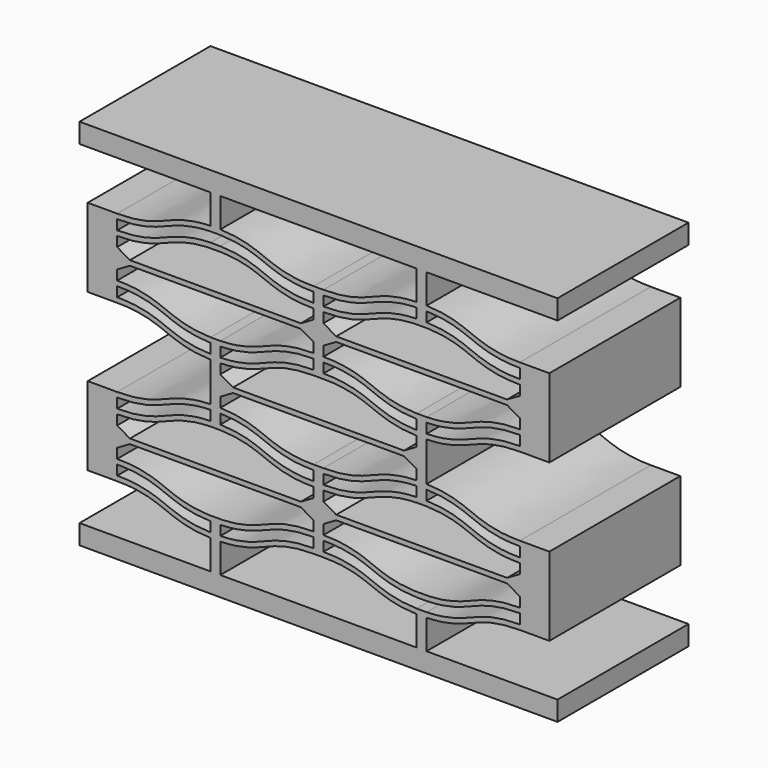
from build123d import *

# Parameters (mm, degrees)
F1_DEPTH = 25


with BuildPart() as f1:
    # F0 (on Front) → F1 (new body)
    with BuildSketch(Plane.XZ):
        with BuildLine():
            add(Edge.make_bspline(
                [(0, 0), (-3.75, 0), (-7.3706402366, -1.4482560946), (-10.9912804731, -2.8965121892), (-14.25, -2.9895365677)],
                knots=[0, 0, 0, 0, 0.5, 0.9655040631, 0.9655040631, 0.9655040631, 0.9655040631], degree=3))
            Line((0, 0), (1.5, 0))
            add(Edge.make_bspline(
                [(15.75, -2.9895365677), (12.4912804731, -2.8965121892), (8.8706402366, -1.4482560946), (5.25, 0), (1.5, 0)],
                knots=[0.0344959369, 0.0344959369, 0.0344959369, 0.0344959369, 0.5, 1, 1, 1, 1], degree=3))
            add(Edge.make_bspline(
                [(16.5, -3), (16.2412804731, -3), (15.9914857187, -2.996430091), (15.75, -2.9895365677)],
                knots=[0, 0, 0, 0, 0.0344959369, 0.0344959369, 0.0344959369, 0.0344959369], degree=3))
            add(Edge.make_bspline(
                [(17.25, -2.9895365677), (17.0085142813, -2.996430091), (16.7587195269, -3), (16.5, -3)],
                knots=[0.9655040631, 0.9655040631, 0.9655040631, 0.9655040631, 1, 1, 1, 1], degree=3))
            add(Edge.make_bspline(
                [(31.5, 0), (27.75, 0), (24.1293597634, -1.4482560946), (20.5087195269, -2.8965121892), (17.25, -2.9895365677)],
                knots=[0, 0, 0, 0, 0.5, 0.9655040631, 0.9655040631, 0.9655040631, 0.9655040631], degree=3))
            Line((31.5, 0), (33, 0))
            Line((33, 0), (36, 0))
            Line((36, 0), (36, 12))
            Line((36, 12), (33, 12))
            Line((33, 12), (31.5, 12))
            add(Edge.make_bspline(
                [(17.25, 14.9895365677), (20.5087195269, 14.8965121892), (24.1293597634, 13.4482560946), (27.75, 12), (31.5, 12)],
                knots=[0.0344959369, 0.0344959369, 0.0344959369, 0.0344959369, 0.5, 1, 1, 1, 1], degree=3))
            add(Edge.make_bspline(
                [(16.5, 15), (16.7587195269, 15), (17.0085142813, 14.996430091), (17.25, 14.9895365677)],
                knots=[0, 0, 0, 0, 0.0344959369, 0.0344959369, 0.0344959369, 0.0344959369], degree=3))
            add(Edge.make_bspline(
                [(15.75, 14.9895365677), (15.9914857187, 14.996430091), (16.2412804731, 15), (16.5, 15)],
                knots=[0.9655040631, 0.9655040631, 0.9655040631, 0.9655040631, 1, 1, 1, 1], degree=3))
            add(Edge.make_bspline(
                [(1.5, 12), (5.25, 12), (8.8706402366, 13.4482560946), (12.4912804731, 14.8965121892), (15.75, 14.9895365677)],
                knots=[0, 0, 0, 0, 0.5, 0.9655040631, 0.9655040631, 0.9655040631, 0.9655040631], degree=3))
            Line((1.5, 12), (0, 12))
            add(Edge.make_bspline(
                [(-14.25, 14.9895365677), (-10.9912804731, 14.8965121892), (-7.3706402366, 13.4482560946), (-3.75, 12), (0, 12)],
                knots=[0.0344959369, 0.0344959369, 0.0344959369, 0.0344959369, 0.5, 1, 1, 1, 1], degree=3))
            add(Edge.make_bspline(
                [(-15, 15), (-14.7412804731, 15), (-14.4914857187, 14.996430091), (-14.25, 14.9895365677)],
                knots=[0, 0, 0, 0, 0.0344959369, 0.0344959369, 0.0344959369, 0.0344959369], degree=3))
            add(Edge.make_bspline(
                [(-15.75, 14.9895365677), (-15.5085142813, 14.996430091), (-15.2587195269, 15), (-15, 15)],
                knots=[0.9655040631, 0.9655040631, 0.9655040631, 0.9655040631, 1, 1, 1, 1], degree=3))
            add(Edge.make_bspline(
                [(-30, 12), (-26.25, 12), (-22.6293597634, 13.4482560946), (-19.0087195269, 14.8965121892), (-15.75, 14.9895365677)],
                knots=[0, 0, 0, 0, 0.5, 0.9655040631, 0.9655040631, 0.9655040631, 0.9655040631], degree=3))
            Line((-30, 12), (-31.5, 12))
            Line((-31.5, 12), (-34.5, 12))
            Line((-34.5, 12), (-34.5, 0))
            Line((-34.5, 0), (-31.5, 0))
            Line((-31.5, 0), (-30, 0))
            add(Edge.make_bspline(
                [(-15.75, -2.9895365677), (-19.0087195269, -2.8965121892), (-22.6293597634, -1.4482560946), (-26.25, 0), (-30, 0)],
                knots=[0.0344959369, 0.0344959369, 0.0344959369, 0.0344959369, 0.5, 1, 1, 1, 1], degree=3))
            add(Edge.make_bspline(
                [(-15, -3), (-15.2587195269, -3), (-15.5085142813, -2.996430091), (-15.75, -2.9895365677)],
                knots=[0, 0, 0, 0, 0.0344959369, 0.0344959369, 0.0344959369, 0.0344959369], degree=3))
            add(Edge.make_bspline(
                [(-14.25, -2.9895365677), (-14.4914857187, -2.996430091), (-14.7412804731, -3), (-15, -3)],
                knots=[0.9655040631, 0.9655040631, 0.9655040631, 0.9655040631, 1, 1, 1, 1], degree=3))
        make_face()
        with BuildLine():
            Line((-30, 0.75), (-30, 2.25))
            add(Edge.make_bspline(
                [(-15.75, -0.7395365677), (-19.0087195269, -0.6465121892), (-22.6293597634, 0.8017439054), (-26.25, 2.25), (-30, 2.25)],
                knots=[0.0344959369, 0.0344959369, 0.0344959369, 0.0344959369, 0.5, 1, 1, 1, 1], degree=3))
            add(Edge.make_bspline(
                [(-15, -0.75), (-15.2587195269, -0.75), (-15.5085142813, -0.746430091), (-15.75, -0.7395365677)],
                knots=[0, 0, 0, 0, 0.0344959369, 0.0344959369, 0.0344959369, 0.0344959369], degree=3))
            add(Edge.make_bspline(
                [(-14.25, -0.7395365677), (-14.4914857187, -0.746430091), (-14.7412804731, -0.75), (-15, -0.75)],
                knots=[0.9655040631, 0.9655040631, 0.9655040631, 0.9655040631, 1, 1, 1, 1], degree=3))
            add(Edge.make_bspline(
                [(0, 2.25), (-3.75, 2.25), (-7.3706402366, 0.8017439054), (-10.9912804731, -0.6465121892), (-14.25, -0.7395365677)],
                knots=[0, 0, 0, 0, 0.5, 0.9655040631, 0.9655040631, 0.9655040631, 0.9655040631], degree=3))
            Line((0, 2.25), (0, 0.75))
            add(Edge.make_bspline(
                [(0, 0.75), (-3.75, 0.75), (-7.3706402366, -0.6982560946), (-10.9912804731, -2.1465121892), (-14.25, -2.2395365677)],
                knots=[0, 0, 0, 0, 0.5, 0.9655040631, 0.9655040631, 0.9655040631, 0.9655040631], degree=3))
            add(Edge.make_bspline(
                [(-14.25, -2.2395365677), (-14.4914857187, -2.246430091), (-14.7412804731, -2.25), (-15, -2.25)],
                knots=[0.9655040631, 0.9655040631, 0.9655040631, 0.9655040631, 1, 1, 1, 1], degree=3))
            add(Edge.make_bspline(
                [(-15, -2.25), (-15.2587195269, -2.25), (-15.5085142813, -2.246430091), (-15.75, -2.2395365677)],
                knots=[0, 0, 0, 0, 0.0344959369, 0.0344959369, 0.0344959369, 0.0344959369], degree=3))
            add(Edge.make_bspline(
                [(-15.75, -2.2395365677), (-19.0087195269, -2.1465121892), (-22.6293597634, -0.6982560946), (-26.25, 0.75), (-30, 0.75)],
                knots=[0.0344959369, 0.0344959369, 0.0344959369, 0.0344959369, 0.5, 1, 1, 1, 1], degree=3))
        make_face(mode=Mode.SUBTRACT)
        with BuildLine():
            Line((-30, 3), (-30, 4.5))
            Line((-30, 4.5), (-28.0514428415, 5.625))
            Line((-28.0514428415, 5.625), (-1.9485571585, 5.625))
            Line((-1.9485571585, 5.625), (0, 4.5))
            Line((0, 4.5), (0, 3))
            add(Edge.make_bspline(
                [(0, 3), (-3.75, 3), (-7.5, 1.5), (-11.25, 0), (-15, 0)],
                knots=[0, 0, 0, 0, 0.5, 1, 1, 1, 1], degree=3))
            add(Edge.make_bspline(
                [(-15, 0), (-18.75, 0), (-22.5, 1.5), (-26.25, 3), (-30, 3)],
                knots=[0, 0, 0, 0, 0.5, 1, 1, 1, 1], degree=3))
        make_face(mode=Mode.SUBTRACT)
        with BuildLine():
            Line((-28.0514428415, 6.375), (-30, 7.5))
            Line((-30, 7.5), (-30, 9))
            add(Edge.make_bspline(
                [(-30, 9), (-26.25, 9), (-22.6293597634, 10.4482560946), (-19.0087195269, 11.8965121892), (-15.75, 11.9895365677)],
                knots=[0, 0, 0, 0, 0.5, 0.9655040631, 0.9655040631, 0.9655040631, 0.9655040631], degree=3))
            add(Edge.make_bspline(
                [(-15.75, 11.9895365677), (-15.5085142813, 11.996430091), (-15.2587195269, 12), (-15, 12)],
                knots=[0.9655040631, 0.9655040631, 0.9655040631, 0.9655040631, 1, 1, 1, 1], degree=3))
            add(Edge.make_bspline(
                [(-15, 12), (-14.7412804731, 12), (-14.4914857187, 11.996430091), (-14.25, 11.9895365677)],
                knots=[0, 0, 0, 0, 0.0344959369, 0.0344959369, 0.0344959369, 0.0344959369], degree=3))
            add(Edge.make_bspline(
                [(-14.25, 11.9895365677), (-10.9912804731, 11.8965121892), (-7.3706402366, 10.4482560946), (-3.75, 9), (0, 9)],
                knots=[0.0344959369, 0.0344959369, 0.0344959369, 0.0344959369, 0.5, 1, 1, 1, 1], degree=3))
            Line((0, 9), (0, 7.5))
            Line((0, 7.5), (-1.9485571585, 6.375))
            Line((-1.9485571585, 6.375), (-15, 6.375))
            Line((-15, 6.375), (-28.0514428415, 6.375))
        make_face(mode=Mode.SUBTRACT)
        with BuildLine():
            add(Edge.make_bspline(
                [(-14.25, 14.2395365677), (-10.9912804731, 14.1465121892), (-7.3706402366, 12.6982560946), (-3.75, 11.25), (0, 11.25)],
                knots=[0.0344959369, 0.0344959369, 0.0344959369, 0.0344959369, 0.5, 1, 1, 1, 1], degree=3))
            Line((0, 11.25), (0, 9.75))
            add(Edge.make_bspline(
                [(-14.25, 12.7395365677), (-10.9912804731, 12.6465121892), (-7.3706402366, 11.1982560946), (-3.75, 9.75), (0, 9.75)],
                knots=[0.0344959369, 0.0344959369, 0.0344959369, 0.0344959369, 0.5, 1, 1, 1, 1], degree=3))
            add(Edge.make_bspline(
                [(-15, 12.75), (-14.7412804731, 12.75), (-14.4914857187, 12.746430091), (-14.25, 12.7395365677)],
                knots=[0, 0, 0, 0, 0.0344959369, 0.0344959369, 0.0344959369, 0.0344959369], degree=3))
            add(Edge.make_bspline(
                [(-15.75, 12.7395365677), (-15.5085142813, 12.746430091), (-15.2587195269, 12.75), (-15, 12.75)],
                knots=[0.9655040631, 0.9655040631, 0.9655040631, 0.9655040631, 1, 1, 1, 1], degree=3))
            add(Edge.make_bspline(
                [(-30, 9.75), (-26.25, 9.75), (-22.6293597634, 11.1982560946), (-19.0087195269, 12.6465121892), (-15.75, 12.7395365677)],
                knots=[0, 0, 0, 0, 0.5, 0.9655040631, 0.9655040631, 0.9655040631, 0.9655040631], degree=3))
            Line((-30, 9.75), (-30, 11.25))
            add(Edge.make_bspline(
                [(-30, 11.25), (-26.25, 11.25), (-22.6293597634, 12.6982560946), (-19.0087195269, 14.1465121892), (-15.75, 14.2395365677)],
                knots=[0, 0, 0, 0, 0.5, 0.9655040631, 0.9655040631, 0.9655040631, 0.9655040631], degree=3))
            add(Edge.make_bspline(
                [(-15.75, 14.2395365677), (-15.5085142813, 14.246430091), (-15.2587195269, 14.25), (-15, 14.25)],
                knots=[0.9655040631, 0.9655040631, 0.9655040631, 0.9655040631, 1, 1, 1, 1], degree=3))
            add(Edge.make_bspline(
                [(-15, 14.25), (-14.7412804731, 14.25), (-14.4914857187, 14.246430091), (-14.25, 14.2395365677)],
                knots=[0, 0, 0, 0, 0.0344959369, 0.0344959369, 0.0344959369, 0.0344959369], degree=3))
        make_face(mode=Mode.SUBTRACT)
        with BuildLine():
            Line((1.5, 0.75), (1.5, 2.25))
            add(Edge.make_bspline(
                [(15.75, -0.7395365677), (12.4912804731, -0.6465121892), (8.8706402366, 0.8017439054), (5.25, 2.25), (1.5, 2.25)],
                knots=[0.0344959369, 0.0344959369, 0.0344959369, 0.0344959369, 0.5, 1, 1, 1, 1], degree=3))
            add(Edge.make_bspline(
                [(16.5, -0.75), (16.2412804731, -0.75), (15.9914857187, -0.746430091), (15.75, -0.7395365677)],
                knots=[0, 0, 0, 0, 0.0344959369, 0.0344959369, 0.0344959369, 0.0344959369], degree=3))
            add(Edge.make_bspline(
                [(17.25, -0.7395365677), (17.0085142813, -0.746430091), (16.7587195269, -0.75), (16.5, -0.75)],
                knots=[0.9655040631, 0.9655040631, 0.9655040631, 0.9655040631, 1, 1, 1, 1], degree=3))
            add(Edge.make_bspline(
                [(31.5, 2.25), (27.75, 2.25), (24.1293597634, 0.8017439054), (20.5087195269, -0.6465121892), (17.25, -0.7395365677)],
                knots=[0, 0, 0, 0, 0.5, 0.9655040631, 0.9655040631, 0.9655040631, 0.9655040631], degree=3))
            Line((31.5, 2.25), (31.5, 0.75))
            add(Edge.make_bspline(
                [(31.5, 0.75), (27.75, 0.75), (24.1293597634, -0.6982560946), (20.5087195269, -2.1465121892), (17.25, -2.2395365677)],
                knots=[0, 0, 0, 0, 0.5, 0.9655040631, 0.9655040631, 0.9655040631, 0.9655040631], degree=3))
            add(Edge.make_bspline(
                [(17.25, -2.2395365677), (17.0085142813, -2.246430091), (16.7587195269, -2.25), (16.5, -2.25)],
                knots=[0.9655040631, 0.9655040631, 0.9655040631, 0.9655040631, 1, 1, 1, 1], degree=3))
            add(Edge.make_bspline(
                [(16.5, -2.25), (16.2412804731, -2.25), (15.9914857187, -2.246430091), (15.75, -2.2395365677)],
                knots=[0, 0, 0, 0, 0.0344959369, 0.0344959369, 0.0344959369, 0.0344959369], degree=3))
            add(Edge.make_bspline(
                [(15.75, -2.2395365677), (12.4912804731, -2.1465121892), (8.8706402366, -0.6982560946), (5.25, 0.75), (1.5, 0.75)],
                knots=[0.0344959369, 0.0344959369, 0.0344959369, 0.0344959369, 0.5, 1, 1, 1, 1], degree=3))
        make_face(mode=Mode.SUBTRACT)
        with BuildLine():
            Line((1.5, 3), (1.5, 4.5))
            Line((1.5, 4.5), (3.4485571585, 5.625))
            Line((3.4485571585, 5.625), (29.5514428415, 5.625))
            Line((29.5514428415, 5.625), (31.5, 4.5))
            Line((31.5, 4.5), (31.5, 3))
            add(Edge.make_bspline(
                [(31.5, 3), (27.75, 3), (24, 1.5), (20.25, 0), (16.5, 0)],
                knots=[0, 0, 0, 0, 0.5, 1, 1, 1, 1], degree=3))
            add(Edge.make_bspline(
                [(16.5, 0), (12.75, 0), (9, 1.5), (5.25, 3), (1.5, 3)],
                knots=[0, 0, 0, 0, 0.5, 1, 1, 1, 1], degree=3))
        make_face(mode=Mode.SUBTRACT)
        with BuildLine():
            Line((3.4485571585, 6.375), (1.5, 7.5))
            Line((1.5, 7.5), (1.5, 9))
            add(Edge.make_bspline(
                [(1.5, 9), (5.25, 9), (8.8706402366, 10.4482560946), (12.4912804731, 11.8965121892), (15.75, 11.9895365677)],
                knots=[0, 0, 0, 0, 0.5, 0.9655040631, 0.9655040631, 0.9655040631, 0.9655040631], degree=3))
            add(Edge.make_bspline(
                [(15.75, 11.9895365677), (15.9914857187, 11.996430091), (16.2412804731, 12), (16.5, 12)],
                knots=[0.9655040631, 0.9655040631, 0.9655040631, 0.9655040631, 1, 1, 1, 1], degree=3))
            add(Edge.make_bspline(
                [(16.5, 12), (16.7587195269, 12), (17.0085142813, 11.996430091), (17.25, 11.9895365677)],
                knots=[0, 0, 0, 0, 0.0344959369, 0.0344959369, 0.0344959369, 0.0344959369], degree=3))
            add(Edge.make_bspline(
                [(17.25, 11.9895365677), (20.5087195269, 11.8965121892), (24.1293597634, 10.4482560946), (27.75, 9), (31.5, 9)],
                knots=[0.0344959369, 0.0344959369, 0.0344959369, 0.0344959369, 0.5, 1, 1, 1, 1], degree=3))
            Line((31.5, 9), (31.5, 7.5))
            Line((31.5, 7.5), (29.5514428415, 6.375))
            Line((29.5514428415, 6.375), (16.5, 6.375))
            Line((16.5, 6.375), (3.4485571585, 6.375))
        make_face(mode=Mode.SUBTRACT)
        with BuildLine():
            Line((1.5, 9.75), (1.5, 11.25))
            add(Edge.make_bspline(
                [(1.5, 11.25), (5.25, 11.25), (8.8706402366, 12.6982560946), (12.4912804731, 14.1465121892), (15.75, 14.2395365677)],
                knots=[0, 0, 0, 0, 0.5, 0.9655040631, 0.9655040631, 0.9655040631, 0.9655040631], degree=3))
            add(Edge.make_bspline(
                [(15.75, 14.2395365677), (15.9914857187, 14.246430091), (16.2412804731, 14.25), (16.5, 14.25)],
                knots=[0.9655040631, 0.9655040631, 0.9655040631, 0.9655040631, 1, 1, 1, 1], degree=3))
            add(Edge.make_bspline(
                [(16.5, 14.25), (16.7587195269, 14.25), (17.0085142813, 14.246430091), (17.25, 14.2395365677)],
                knots=[0, 0, 0, 0, 0.0344959369, 0.0344959369, 0.0344959369, 0.0344959369], degree=3))
            add(Edge.make_bspline(
                [(17.25, 14.2395365677), (20.5087195269, 14.1465121892), (24.1293597634, 12.6982560946), (27.75, 11.25), (31.5, 11.25)],
                knots=[0.0344959369, 0.0344959369, 0.0344959369, 0.0344959369, 0.5, 1, 1, 1, 1], degree=3))
            Line((31.5, 11.25), (31.5, 9.75))
            add(Edge.make_bspline(
                [(17.25, 12.7395365677), (20.5087195269, 12.6465121892), (24.1293597634, 11.1982560946), (27.75, 9.75), (31.5, 9.75)],
                knots=[0.0344959369, 0.0344959369, 0.0344959369, 0.0344959369, 0.5, 1, 1, 1, 1], degree=3))
            add(Edge.make_bspline(
                [(16.5, 12.75), (16.7587195269, 12.75), (17.0085142813, 12.746430091), (17.25, 12.7395365677)],
                knots=[0, 0, 0, 0, 0.0344959369, 0.0344959369, 0.0344959369, 0.0344959369], degree=3))
            add(Edge.make_bspline(
                [(15.75, 12.7395365677), (15.9914857187, 12.746430091), (16.2412804731, 12.75), (16.5, 12.75)],
                knots=[0.9655040631, 0.9655040631, 0.9655040631, 0.9655040631, 1, 1, 1, 1], degree=3))
            add(Edge.make_bspline(
                [(1.5, 9.75), (5.25, 9.75), (8.8706402366, 11.1982560946), (12.4912804731, 12.6465121892), (15.75, 12.7395365677)],
                knots=[0, 0, 0, 0, 0.5, 0.9655040631, 0.9655040631, 0.9655040631, 0.9655040631], degree=3))
        make_face(mode=Mode.SUBTRACT)
        with BuildLine():
            add(Edge.make_bspline(
                [(-15.75, 20.9895365677), (-19.0087195269, 21.0825609462), (-22.6293597634, 22.5308170408), (-26.25, 23.9790731355), (-30, 23.9790731355)],
                knots=[0.0344959369, 0.0344959369, 0.0344959369, 0.0344959369, 0.5, 1, 1, 1, 1], degree=3))
            add(Edge.make_bspline(
                [(-15, 20.9790731355), (-15.2587195269, 20.9790731355), (-15.5085142813, 20.9826430445), (-15.75, 20.9895365677)],
                knots=[0, 0, 0, 0, 0.0344959369, 0.0344959369, 0.0344959369, 0.0344959369], degree=3))
            add(Edge.make_bspline(
                [(-14.25, 20.9895365677), (-14.4914857187, 20.9826430445), (-14.7412804731, 20.9790731355), (-15, 20.9790731355)],
                knots=[0.9655040631, 0.9655040631, 0.9655040631, 0.9655040631, 1, 1, 1, 1], degree=3))
            add(Edge.make_bspline(
                [(0, 23.9790731355), (-3.75, 23.9790731355), (-7.3706402366, 22.5308170408), (-10.9912804731, 21.0825609462), (-14.25, 20.9895365677)],
                knots=[0, 0, 0, 0, 0.5, 0.9655040631, 0.9655040631, 0.9655040631, 0.9655040631], degree=3))
            Line((0, 23.9790731355), (1.5, 23.9790731355))
            add(Edge.make_bspline(
                [(15.75, 20.9895365677), (12.4912804731, 21.0825609462), (8.8706402366, 22.5308170408), (5.25, 23.9790731355), (1.5, 23.9790731355)],
                knots=[0.0344959369, 0.0344959369, 0.0344959369, 0.0344959369, 0.5, 1, 1, 1, 1], degree=3))
            add(Edge.make_bspline(
                [(16.5, 20.9790731355), (16.2412804731, 20.9790731355), (15.9914857187, 20.9826430445), (15.75, 20.9895365677)],
                knots=[0, 0, 0, 0, 0.0344959369, 0.0344959369, 0.0344959369, 0.0344959369], degree=3))
            add(Edge.make_bspline(
                [(17.25, 20.9895365677), (17.0085142813, 20.9826430445), (16.7587195269, 20.9790731355), (16.5, 20.9790731355)],
                knots=[0.9655040631, 0.9655040631, 0.9655040631, 0.9655040631, 1, 1, 1, 1], degree=3))
            add(Edge.make_bspline(
                [(31.5, 23.9790731355), (27.75, 23.9790731355), (24.1293597634, 22.5308170408), (20.5087195269, 21.0825609462), (17.25, 20.9895365677)],
                knots=[0, 0, 0, 0, 0.5, 0.9655040631, 0.9655040631, 0.9655040631, 0.9655040631], degree=3))
            Line((31.5, 23.9790731355), (33, 23.9790731355))
            Line((33, 23.9790731355), (36, 23.9790731355))
            Line((36, 23.9790731355), (36, 35.9790731355))
            Line((36, 35.9790731355), (33, 35.9790731355))
            Line((33, 35.9790731355), (31.5, 35.9790731355))
            add(Edge.make_bspline(
                [(17.25, 38.9686097032), (20.5087195269, 38.8755853247), (24.1293597634, 37.4273292301), (27.75, 35.9790731355), (31.5, 35.9790731355)],
                knots=[0.0344959369, 0.0344959369, 0.0344959369, 0.0344959369, 0.5, 1, 1, 1, 1], degree=3))
            add(Edge.make_bspline(
                [(16.5, 38.9790731355), (16.7587195269, 38.9790731355), (17.0085142813, 38.9755032265), (17.25, 38.9686097032)],
                knots=[0, 0, 0, 0, 0.0344959369, 0.0344959369, 0.0344959369, 0.0344959369], degree=3))
            add(Edge.make_bspline(
                [(15.75, 38.9686097032), (15.9914857187, 38.9755032265), (16.2412804731, 38.9790731355), (16.5, 38.9790731355)],
                knots=[0.9655040631, 0.9655040631, 0.9655040631, 0.9655040631, 1, 1, 1, 1], degree=3))
            add(Edge.make_bspline(
                [(1.5, 35.9790731355), (5.25, 35.9790731355), (8.8706402366, 37.4273292301), (12.4912804731, 38.8755853247), (15.75, 38.9686097032)],
                knots=[0, 0, 0, 0, 0.5, 0.9655040631, 0.9655040631, 0.9655040631, 0.9655040631], degree=3))
            Line((1.5, 35.9790731355), (0, 35.9790731355))
            add(Edge.make_bspline(
                [(-14.25, 38.9686097032), (-10.9912804731, 38.8755853247), (-7.3706402366, 37.4273292301), (-3.75, 35.9790731355), (0, 35.9790731355)],
                knots=[0.0344959369, 0.0344959369, 0.0344959369, 0.0344959369, 0.5, 1, 1, 1, 1], degree=3))
            add(Edge.make_bspline(
                [(-15, 38.9790731355), (-14.7412804731, 38.9790731355), (-14.4914857187, 38.9755032265), (-14.25, 38.9686097032)],
                knots=[0, 0, 0, 0, 0.0344959369, 0.0344959369, 0.0344959369, 0.0344959369], degree=3))
            add(Edge.make_bspline(
                [(-15.75, 38.9686097032), (-15.5085142813, 38.9755032265), (-15.2587195269, 38.9790731355), (-15, 38.9790731355)],
                knots=[0.9655040631, 0.9655040631, 0.9655040631, 0.9655040631, 1, 1, 1, 1], degree=3))
            add(Edge.make_bspline(
                [(-30, 35.9790731355), (-26.25, 35.9790731355), (-22.6293597634, 37.4273292301), (-19.0087195269, 38.8755853247), (-15.75, 38.9686097032)],
                knots=[0, 0, 0, 0, 0.5, 0.9655040631, 0.9655040631, 0.9655040631, 0.9655040631], degree=3))
            Line((-30, 35.9790731355), (-31.5, 35.9790731355))
            Line((-31.5, 35.9790731355), (-34.5, 35.9790731355))
            Line((-34.5, 35.9790731355), (-34.5, 23.9790731355))
            Line((-34.5, 23.9790731355), (-31.5, 23.9790731355))
            Line((-31.5, 23.9790731355), (-30, 23.9790731355))
        make_face()
        with BuildLine():
            add(Edge.make_bspline(
                [(-15, 21.7290731355), (-15.2587195269, 21.7290731355), (-15.5085142813, 21.7326430445), (-15.75, 21.7395365677)],
                knots=[0, 0, 0, 0, 0.0344959369, 0.0344959369, 0.0344959369, 0.0344959369], degree=3))
            add(Edge.make_bspline(
                [(-15.75, 21.7395365677), (-19.0087195269, 21.8325609462), (-22.6293597634, 23.2808170408), (-26.25, 24.7290731355), (-30, 24.7290731355)],
                knots=[0.0344959369, 0.0344959369, 0.0344959369, 0.0344959369, 0.5, 1, 1, 1, 1], degree=3))
            Line((-30, 24.7290731355), (-30, 26.2290731355))
            add(Edge.make_bspline(
                [(-15.75, 23.2395365677), (-19.0087195269, 23.3325609462), (-22.6293597634, 24.7808170408), (-26.25, 26.2290731355), (-30, 26.2290731355)],
                knots=[0.0344959369, 0.0344959369, 0.0344959369, 0.0344959369, 0.5, 1, 1, 1, 1], degree=3))
            add(Edge.make_bspline(
                [(-15, 23.2290731355), (-15.2587195269, 23.2290731355), (-15.5085142813, 23.2326430445), (-15.75, 23.2395365677)],
                knots=[0, 0, 0, 0, 0.0344959369, 0.0344959369, 0.0344959369, 0.0344959369], degree=3))
            add(Edge.make_bspline(
                [(-14.25, 23.2395365677), (-14.4914857187, 23.2326430445), (-14.7412804731, 23.2290731355), (-15, 23.2290731355)],
                knots=[0.9655040631, 0.9655040631, 0.9655040631, 0.9655040631, 1, 1, 1, 1], degree=3))
            add(Edge.make_bspline(
                [(0, 26.2290731355), (-3.75, 26.2290731355), (-7.3706402366, 24.7808170408), (-10.9912804731, 23.3325609462), (-14.25, 23.2395365677)],
                knots=[0, 0, 0, 0, 0.5, 0.9655040631, 0.9655040631, 0.9655040631, 0.9655040631], degree=3))
            Line((0, 26.2290731355), (0, 24.7290731355))
            add(Edge.make_bspline(
                [(0, 24.7290731355), (-3.75, 24.7290731355), (-7.3706402366, 23.2808170408), (-10.9912804731, 21.8325609462), (-14.25, 21.7395365677)],
                knots=[0, 0, 0, 0, 0.5, 0.9655040631, 0.9655040631, 0.9655040631, 0.9655040631], degree=3))
            add(Edge.make_bspline(
                [(-14.25, 21.7395365677), (-14.4914857187, 21.7326430445), (-14.7412804731, 21.7290731355), (-15, 21.7290731355)],
                knots=[0.9655040631, 0.9655040631, 0.9655040631, 0.9655040631, 1, 1, 1, 1], degree=3))
        make_face(mode=Mode.SUBTRACT)
        with BuildLine():
            add(Edge.make_bspline(
                [(-15, 23.9790731355), (-15.2587195269, 23.9790731355), (-15.5085142813, 23.9826430445), (-15.75, 23.9895365677)],
                knots=[0, 0, 0, 0, 0.0344959369, 0.0344959369, 0.0344959369, 0.0344959369], degree=3))
            add(Edge.make_bspline(
                [(-15.75, 23.9895365677), (-19.0087195269, 24.0825609462), (-22.6293597634, 25.5308170408), (-26.25, 26.9790731355), (-30, 26.9790731355)],
                knots=[0.0344959369, 0.0344959369, 0.0344959369, 0.0344959369, 0.5, 1, 1, 1, 1], degree=3))
            Line((-30, 26.9790731355), (-30, 28.4790731355))
            Line((-30, 28.4790731355), (-28.0514428415, 29.6040731355))
            Line((-28.0514428415, 29.6040731355), (-1.9485571585, 29.6040731355))
            Line((-1.9485571585, 29.6040731355), (0, 28.4790731355))
            Line((0, 28.4790731355), (0, 26.9790731355))
            add(Edge.make_bspline(
                [(0, 26.9790731355), (-3.75, 26.9790731355), (-7.3706402366, 25.5308170408), (-10.9912804731, 24.0825609462), (-14.25, 23.9895365677)],
                knots=[0, 0, 0, 0, 0.5, 0.9655040631, 0.9655040631, 0.9655040631, 0.9655040631], degree=3))
            add(Edge.make_bspline(
                [(-14.25, 23.9895365677), (-14.4914857187, 23.9826430445), (-14.7412804731, 23.9790731355), (-15, 23.9790731355)],
                knots=[0.9655040631, 0.9655040631, 0.9655040631, 0.9655040631, 1, 1, 1, 1], degree=3))
        make_face(mode=Mode.SUBTRACT)
        with BuildLine():
            Line((-28.0514428415, 30.3540731355), (-30, 31.4790731355))
            Line((-30, 31.4790731355), (-30, 32.9790731355))
            add(Edge.make_bspline(
                [(-30, 32.9790731355), (-26.25, 32.9790731355), (-22.5, 34.4790731355), (-18.75, 35.9790731355), (-15, 35.9790731355)],
                knots=[0, 0, 0, 0, 0.5, 1, 1, 1, 1], degree=3))
            add(Edge.make_bspline(
                [(-15, 35.9790731355), (-11.25, 35.9790731355), (-7.5, 34.4790731355), (-3.75, 32.9790731355), (0, 32.9790731355)],
                knots=[0, 0, 0, 0, 0.5, 1, 1, 1, 1], degree=3))
            Line((0, 32.9790731355), (0, 31.4790731355))
            Line((0, 31.4790731355), (-1.9485571585, 30.3540731355))
            Line((-1.9485571585, 30.3540731355), (-15, 30.3540731355))
            Line((-15, 30.3540731355), (-28.0514428415, 30.3540731355))
        make_face(mode=Mode.SUBTRACT)
        with BuildLine():
            Line((-30, 33.7290731355), (-30, 35.2290731355))
            add(Edge.make_bspline(
                [(-30, 35.2290731355), (-26.25, 35.2290731355), (-22.6293597634, 36.6773292301), (-19.0087195269, 38.1255853247), (-15.75, 38.2186097032)],
                knots=[0, 0, 0, 0, 0.5, 0.9655040631, 0.9655040631, 0.9655040631, 0.9655040631], degree=3))
            add(Edge.make_bspline(
                [(-15.75, 38.2186097032), (-15.5085142813, 38.2255032265), (-15.2587195269, 38.2290731355), (-15, 38.2290731355)],
                knots=[0.9655040631, 0.9655040631, 0.9655040631, 0.9655040631, 1, 1, 1, 1], degree=3))
            add(Edge.make_bspline(
                [(-15, 38.2290731355), (-14.7412804731, 38.2290731355), (-14.4914857187, 38.2255032265), (-14.25, 38.2186097032)],
                knots=[0, 0, 0, 0, 0.0344959369, 0.0344959369, 0.0344959369, 0.0344959369], degree=3))
            add(Edge.make_bspline(
                [(-14.25, 38.2186097032), (-10.9912804731, 38.1255853247), (-7.3706402366, 36.6773292301), (-3.75, 35.2290731355), (0, 35.2290731355)],
                knots=[0.0344959369, 0.0344959369, 0.0344959369, 0.0344959369, 0.5, 1, 1, 1, 1], degree=3))
            Line((0, 35.2290731355), (0, 33.7290731355))
            add(Edge.make_bspline(
                [(-14.25, 36.7186097032), (-10.9912804731, 36.6255853247), (-7.3706402366, 35.1773292301), (-3.75, 33.7290731355), (0, 33.7290731355)],
                knots=[0.0344959369, 0.0344959369, 0.0344959369, 0.0344959369, 0.5, 1, 1, 1, 1], degree=3))
            add(Edge.make_bspline(
                [(-15, 36.7290731355), (-14.7412804731, 36.7290731355), (-14.4914857187, 36.7255032265), (-14.25, 36.7186097032)],
                knots=[0, 0, 0, 0, 0.0344959369, 0.0344959369, 0.0344959369, 0.0344959369], degree=3))
            add(Edge.make_bspline(
                [(-15.75, 36.7186097032), (-15.5085142813, 36.7255032265), (-15.2587195269, 36.7290731355), (-15, 36.7290731355)],
                knots=[0.9655040631, 0.9655040631, 0.9655040631, 0.9655040631, 1, 1, 1, 1], degree=3))
            add(Edge.make_bspline(
                [(-30, 33.7290731355), (-26.25, 33.7290731355), (-22.6293597634, 35.1773292301), (-19.0087195269, 36.6255853247), (-15.75, 36.7186097032)],
                knots=[0, 0, 0, 0, 0.5, 0.9655040631, 0.9655040631, 0.9655040631, 0.9655040631], degree=3))
        make_face(mode=Mode.SUBTRACT)
        with BuildLine():
            add(Edge.make_bspline(
                [(31.5, 24.7290731355), (27.75, 24.7290731355), (24.1293597634, 23.2808170408), (20.5087195269, 21.8325609462), (17.25, 21.7395365677)],
                knots=[0, 0, 0, 0, 0.5, 0.9655040631, 0.9655040631, 0.9655040631, 0.9655040631], degree=3))
            add(Edge.make_bspline(
                [(17.25, 21.7395365677), (17.0085142813, 21.7326430445), (16.7587195269, 21.7290731355), (16.5, 21.7290731355)],
                knots=[0.9655040631, 0.9655040631, 0.9655040631, 0.9655040631, 1, 1, 1, 1], degree=3))
            add(Edge.make_bspline(
                [(16.5, 21.7290731355), (16.2412804731, 21.7290731355), (15.9914857187, 21.7326430445), (15.75, 21.7395365677)],
                knots=[0, 0, 0, 0, 0.0344959369, 0.0344959369, 0.0344959369, 0.0344959369], degree=3))
            add(Edge.make_bspline(
                [(15.75, 21.7395365677), (12.4912804731, 21.8325609462), (8.8706402366, 23.2808170408), (5.25, 24.7290731355), (1.5, 24.7290731355)],
                knots=[0.0344959369, 0.0344959369, 0.0344959369, 0.0344959369, 0.5, 1, 1, 1, 1], degree=3))
            Line((1.5, 24.7290731355), (1.5, 26.2290731355))
            add(Edge.make_bspline(
                [(15.75, 23.2395365677), (12.4912804731, 23.3325609462), (8.8706402366, 24.7808170408), (5.25, 26.2290731355), (1.5, 26.2290731355)],
                knots=[0.0344959369, 0.0344959369, 0.0344959369, 0.0344959369, 0.5, 1, 1, 1, 1], degree=3))
            add(Edge.make_bspline(
                [(16.5, 23.2290731355), (16.2412804731, 23.2290731355), (15.9914857187, 23.2326430445), (15.75, 23.2395365677)],
                knots=[0, 0, 0, 0, 0.0344959369, 0.0344959369, 0.0344959369, 0.0344959369], degree=3))
            add(Edge.make_bspline(
                [(17.25, 23.2395365677), (17.0085142813, 23.2326430445), (16.7587195269, 23.2290731355), (16.5, 23.2290731355)],
                knots=[0.9655040631, 0.9655040631, 0.9655040631, 0.9655040631, 1, 1, 1, 1], degree=3))
            add(Edge.make_bspline(
                [(31.5, 26.2290731355), (27.75, 26.2290731355), (24.1293597634, 24.7808170408), (20.5087195269, 23.3325609462), (17.25, 23.2395365677)],
                knots=[0, 0, 0, 0, 0.5, 0.9655040631, 0.9655040631, 0.9655040631, 0.9655040631], degree=3))
            Line((31.5, 26.2290731355), (31.5, 24.7290731355))
        make_face(mode=Mode.SUBTRACT)
        with BuildLine():
            add(Edge.make_bspline(
                [(31.5, 26.9790731355), (27.75, 26.9790731355), (24.1293597634, 25.5308170408), (20.5087195269, 24.0825609462), (17.25, 23.9895365677)],
                knots=[0, 0, 0, 0, 0.5, 0.9655040631, 0.9655040631, 0.9655040631, 0.9655040631], degree=3))
            add(Edge.make_bspline(
                [(17.25, 23.9895365677), (17.0085142813, 23.9826430445), (16.7587195269, 23.9790731355), (16.5, 23.9790731355)],
                knots=[0.9655040631, 0.9655040631, 0.9655040631, 0.9655040631, 1, 1, 1, 1], degree=3))
            add(Edge.make_bspline(
                [(16.5, 23.9790731355), (16.2412804731, 23.9790731355), (15.9914857187, 23.9826430445), (15.75, 23.9895365677)],
                knots=[0, 0, 0, 0, 0.0344959369, 0.0344959369, 0.0344959369, 0.0344959369], degree=3))
            add(Edge.make_bspline(
                [(15.75, 23.9895365677), (12.4912804731, 24.0825609462), (8.8706402366, 25.5308170408), (5.25, 26.9790731355), (1.5, 26.9790731355)],
                knots=[0.0344959369, 0.0344959369, 0.0344959369, 0.0344959369, 0.5, 1, 1, 1, 1], degree=3))
            Line((1.5, 26.9790731355), (1.5, 28.4790731355))
            Line((1.5, 28.4790731355), (3.4485571585, 29.6040731355))
            Line((3.4485571585, 29.6040731355), (29.5514428415, 29.6040731355))
            Line((29.5514428415, 29.6040731355), (31.5, 28.4790731355))
            Line((31.5, 28.4790731355), (31.5, 26.9790731355))
        make_face(mode=Mode.SUBTRACT)
        with BuildLine():
            Line((3.4485571585, 30.3540731355), (1.5, 31.4790731355))
            Line((1.5, 31.4790731355), (1.5, 32.9790731355))
            add(Edge.make_bspline(
                [(1.5, 32.9790731355), (5.25, 32.9790731355), (9, 34.4790731355), (12.75, 35.9790731355), (16.5, 35.9790731355)],
                knots=[0, 0, 0, 0, 0.5, 1, 1, 1, 1], degree=3))
            add(Edge.make_bspline(
                [(16.5, 35.9790731355), (20.25, 35.9790731355), (24, 34.4790731355), (27.75, 32.9790731355), (31.5, 32.9790731355)],
                knots=[0, 0, 0, 0, 0.5, 1, 1, 1, 1], degree=3))
            Line((31.5, 32.9790731355), (31.5, 31.4790731355))
            Line((31.5, 31.4790731355), (29.5514428415, 30.3540731355))
            Line((29.5514428415, 30.3540731355), (16.5, 30.3540731355))
            Line((16.5, 30.3540731355), (3.4485571585, 30.3540731355))
        make_face(mode=Mode.SUBTRACT)
        with BuildLine():
            Line((1.5, 33.7290731355), (1.5, 35.2290731355))
            add(Edge.make_bspline(
                [(1.5, 35.2290731355), (5.25, 35.2290731355), (8.8706402366, 36.6773292301), (12.4912804731, 38.1255853247), (15.75, 38.2186097032)],
                knots=[0, 0, 0, 0, 0.5, 0.9655040631, 0.9655040631, 0.9655040631, 0.9655040631], degree=3))
            add(Edge.make_bspline(
                [(15.75, 38.2186097032), (15.9914857187, 38.2255032265), (16.2412804731, 38.2290731355), (16.5, 38.2290731355)],
                knots=[0.9655040631, 0.9655040631, 0.9655040631, 0.9655040631, 1, 1, 1, 1], degree=3))
            add(Edge.make_bspline(
                [(16.5, 38.2290731355), (16.7587195269, 38.2290731355), (17.0085142813, 38.2255032265), (17.25, 38.2186097032)],
                knots=[0, 0, 0, 0, 0.0344959369, 0.0344959369, 0.0344959369, 0.0344959369], degree=3))
            add(Edge.make_bspline(
                [(17.25, 38.2186097032), (20.5087195269, 38.1255853247), (24.1293597634, 36.6773292301), (27.75, 35.2290731355), (31.5, 35.2290731355)],
                knots=[0.0344959369, 0.0344959369, 0.0344959369, 0.0344959369, 0.5, 1, 1, 1, 1], degree=3))
            Line((31.5, 35.2290731355), (31.5, 33.7290731355))
            add(Edge.make_bspline(
                [(17.25, 36.7186097032), (20.5087195269, 36.6255853247), (24.1293597634, 35.1773292301), (27.75, 33.7290731355), (31.5, 33.7290731355)],
                knots=[0.0344959369, 0.0344959369, 0.0344959369, 0.0344959369, 0.5, 1, 1, 1, 1], degree=3))
            add(Edge.make_bspline(
                [(16.5, 36.7290731355), (16.7587195269, 36.7290731355), (17.0085142813, 36.7255032265), (17.25, 36.7186097032)],
                knots=[0, 0, 0, 0, 0.0344959369, 0.0344959369, 0.0344959369, 0.0344959369], degree=3))
            add(Edge.make_bspline(
                [(15.75, 36.7186097032), (15.9914857187, 36.7255032265), (16.2412804731, 36.7290731355), (16.5, 36.7290731355)],
                knots=[0.9655040631, 0.9655040631, 0.9655040631, 0.9655040631, 1, 1, 1, 1], degree=3))
            add(Edge.make_bspline(
                [(1.5, 33.7290731355), (5.25, 33.7290731355), (8.8706402366, 35.1773292301), (12.4912804731, 36.6255853247), (15.75, 36.7186097032)],
                knots=[0, 0, 0, 0, 0.5, 0.9655040631, 0.9655040631, 0.9655040631, 0.9655040631], degree=3))
        make_face(mode=Mode.SUBTRACT)
        with BuildLine():
            Line((-14.25, -7.4895365677), (-14.25, -2.9895365677))
            add(Edge.make_bspline(
                [(-14.25, -2.9895365677), (-14.4914857187, -2.996430091), (-14.7412804731, -3), (-15, -3)],
                knots=[0.9655040631, 0.9655040631, 0.9655040631, 0.9655040631, 1, 1, 1, 1], degree=3))
            add(Edge.make_bspline(
                [(-15, -3), (-15.2587195269, -3), (-15.5085142813, -2.996430091), (-15.75, -2.9895365677)],
                knots=[0, 0, 0, 0, 0.0344959369, 0.0344959369, 0.0344959369, 0.0344959369], degree=3))
            Line((-15.75, -2.9895365677), (-15.75, -7.4895365677))
            Line((-15.75, -7.4895365677), (-35.75, -7.4895365677))
            Line((-35.75, -7.4895365677), (-35.75, -10.4895365677))
            Line((-35.75, -10.4895365677), (37.25, -10.4895365677))
            Line((37.25, -10.4895365677), (37.25, -7.4895365677))
            Line((37.25, -7.4895365677), (17.25, -7.4895365677))
            Line((17.25, -7.4895365677), (17.25, -2.9895365677))
            add(Edge.make_bspline(
                [(17.25, -2.9895365677), (17.0085142813, -2.996430091), (16.7587195269, -3), (16.5, -3)],
                knots=[0.9655040631, 0.9655040631, 0.9655040631, 0.9655040631, 1, 1, 1, 1], degree=3))
            add(Edge.make_bspline(
                [(16.5, -3), (16.2412804731, -3), (15.9914857187, -2.996430091), (15.75, -2.9895365677)],
                knots=[0, 0, 0, 0, 0.0344959369, 0.0344959369, 0.0344959369, 0.0344959369], degree=3))
            Line((15.75, -2.9895365677), (15.75, -7.4895365677))
            Line((15.75, -7.4895365677), (-14.25, -7.4895365677))
        make_face()
        with BuildLine():
            Line((-15.75, 43.4686097032), (-15.75, 38.9686097032))
            add(Edge.make_bspline(
                [(-15.75, 38.9686097032), (-15.5085142813, 38.9755032265), (-15.2587195269, 38.9790731355), (-15, 38.9790731355)],
                knots=[0.9655040631, 0.9655040631, 0.9655040631, 0.9655040631, 1, 1, 1, 1], degree=3))
            add(Edge.make_bspline(
                [(-15, 38.9790731355), (-14.7412804731, 38.9790731355), (-14.4914857187, 38.9755032265), (-14.25, 38.9686097032)],
                knots=[0, 0, 0, 0, 0.0344959369, 0.0344959369, 0.0344959369, 0.0344959369], degree=3))
            Line((-14.25, 38.9686097032), (-14.25, 43.4686097032))
            Line((-14.25, 43.4686097032), (15.75, 43.4686097032))
            Line((15.75, 43.4686097032), (15.75, 38.9686097032))
            add(Edge.make_bspline(
                [(15.75, 38.9686097032), (15.9914857187, 38.9755032265), (16.2412804731, 38.9790731355), (16.5, 38.9790731355)],
                knots=[0.9655040631, 0.9655040631, 0.9655040631, 0.9655040631, 1, 1, 1, 1], degree=3))
            add(Edge.make_bspline(
                [(16.5, 38.9790731355), (16.7587195269, 38.9790731355), (17.0085142813, 38.9755032265), (17.25, 38.9686097032)],
                knots=[0, 0, 0, 0, 0.0344959369, 0.0344959369, 0.0344959369, 0.0344959369], degree=3))
            Line((17.25, 38.9686097032), (17.25, 43.4686097032))
            Line((17.25, 43.4686097032), (37.25, 43.4686097032))
            Line((37.25, 43.4686097032), (37.25, 46.4686097032))
            Line((37.25, 46.4686097032), (-35.75, 46.4686097032))
            Line((-35.75, 46.4686097032), (-35.75, 43.4686097032))
            Line((-35.75, 43.4686097032), (-15.75, 43.4686097032))
        make_face()
        with BuildLine():
            Line((-15.75, 16.4895365677), (-15.75, 14.9895365677))
            add(Edge.make_bspline(
                [(-15.75, 14.9895365677), (-15.5085142813, 14.996430091), (-15.2587195269, 15), (-15, 15)],
                knots=[0.9655040631, 0.9655040631, 0.9655040631, 0.9655040631, 1, 1, 1, 1], degree=3))
            add(Edge.make_bspline(
                [(-15, 15), (-14.7412804731, 15), (-14.4914857187, 14.996430091), (-14.25, 14.9895365677)],
                knots=[0, 0, 0, 0, 0.0344959369, 0.0344959369, 0.0344959369, 0.0344959369], degree=3))
            Line((-14.25, 14.9895365677), (-14.25, 16.4895365677))
            Line((-14.25, 16.4895365677), (-12.3014428415, 17.6145365677))
            Line((-12.3014428415, 17.6145365677), (13.8014428415, 17.6145365677))
            Line((13.8014428415, 17.6145365677), (15.75, 16.4895365677))
            Line((15.75, 16.4895365677), (15.75, 14.9895365677))
            add(Edge.make_bspline(
                [(15.75, 14.9895365677), (15.9914857187, 14.996430091), (16.2412804731, 15), (16.5, 15)],
                knots=[0.9655040631, 0.9655040631, 0.9655040631, 0.9655040631, 1, 1, 1, 1], degree=3))
            add(Edge.make_bspline(
                [(16.5, 15), (16.7587195269, 15), (17.0085142813, 14.996430091), (17.25, 14.9895365677)],
                knots=[0, 0, 0, 0, 0.0344959369, 0.0344959369, 0.0344959369, 0.0344959369], degree=3))
            Line((17.25, 14.9895365677), (17.25, 16.4895365677))
            Line((17.25, 16.4895365677), (17.25, 19.4895365677))
            Line((17.25, 19.4895365677), (15.75, 19.4895365677))
            Line((15.75, 19.4895365677), (13.8014428415, 18.3645365677))
            Line((13.8014428415, 18.3645365677), (0.75, 18.3645365677))
            Line((0.75, 18.3645365677), (-12.3014428415, 18.3645365677))
            Line((-12.3014428415, 18.3645365677), (-14.25, 19.4895365677))
            Line((-14.25, 19.4895365677), (-14.25, 20.9895365677))
            add(Edge.make_bspline(
                [(-14.25, 20.9895365677), (-14.4914857187, 20.9826430445), (-14.7412804731, 20.9790731355), (-15, 20.9790731355)],
                knots=[0.9655040631, 0.9655040631, 0.9655040631, 0.9655040631, 1, 1, 1, 1], degree=3))
            add(Edge.make_bspline(
                [(-15, 20.9790731355), (-15.2587195269, 20.9790731355), (-15.5085142813, 20.9826430445), (-15.75, 20.9895365677)],
                knots=[0, 0, 0, 0, 0.0344959369, 0.0344959369, 0.0344959369, 0.0344959369], degree=3))
            Line((-15.75, 20.9895365677), (-15.75, 19.4895365677))
            Line((-15.75, 19.4895365677), (-15.75, 16.4895365677))
        make_face()
        with BuildLine():
            Line((-14.25, 12.7395365677), (-14.25, 14.2395365677))
            add(Edge.make_bspline(
                [(-15, 14.25), (-14.7412804731, 14.25), (-14.4914857187, 14.246430091), (-14.25, 14.2395365677)],
                knots=[0, 0, 0, 0, 0.0344959369, 0.0344959369, 0.0344959369, 0.0344959369], degree=3))
            add(Edge.make_bspline(
                [(-15.75, 14.2395365677), (-15.5085142813, 14.246430091), (-15.2587195269, 14.25), (-15, 14.25)],
                knots=[0.9655040631, 0.9655040631, 0.9655040631, 0.9655040631, 1, 1, 1, 1], degree=3))
            Line((-15.75, 14.2395365677), (-15.75, 12.7395365677))
            add(Edge.make_bspline(
                [(-15.75, 12.7395365677), (-15.5085142813, 12.746430091), (-15.2587195269, 12.75), (-15, 12.75)],
                knots=[0.9655040631, 0.9655040631, 0.9655040631, 0.9655040631, 1, 1, 1, 1], degree=3))
            add(Edge.make_bspline(
                [(-15, 12.75), (-14.7412804731, 12.75), (-14.4914857187, 12.746430091), (-14.25, 12.7395365677)],
                knots=[0, 0, 0, 0, 0.0344959369, 0.0344959369, 0.0344959369, 0.0344959369], degree=3))
        make_face()
        with BuildLine():
            Line((-15.75, 23.2395365677), (-15.75, 21.7395365677))
            add(Edge.make_bspline(
                [(-15, 21.7290731355), (-15.2587195269, 21.7290731355), (-15.5085142813, 21.7326430445), (-15.75, 21.7395365677)],
                knots=[0, 0, 0, 0, 0.0344959369, 0.0344959369, 0.0344959369, 0.0344959369], degree=3))
            add(Edge.make_bspline(
                [(-14.25, 21.7395365677), (-14.4914857187, 21.7326430445), (-14.7412804731, 21.7290731355), (-15, 21.7290731355)],
                knots=[0.9655040631, 0.9655040631, 0.9655040631, 0.9655040631, 1, 1, 1, 1], degree=3))
            Line((-14.25, 21.7395365677), (-14.25, 23.2395365677))
            add(Edge.make_bspline(
                [(-14.25, 23.2395365677), (-14.4914857187, 23.2326430445), (-14.7412804731, 23.2290731355), (-15, 23.2290731355)],
                knots=[0.9655040631, 0.9655040631, 0.9655040631, 0.9655040631, 1, 1, 1, 1], degree=3))
            add(Edge.make_bspline(
                [(-15, 23.2290731355), (-15.2587195269, 23.2290731355), (-15.5085142813, 23.2326430445), (-15.75, 23.2395365677)],
                knots=[0, 0, 0, 0, 0.0344959369, 0.0344959369, 0.0344959369, 0.0344959369], degree=3))
        make_face()
        with BuildLine():
            add(Edge.make_bspline(
                [(17.25, 21.7395365677), (17.0085142813, 21.7326430445), (16.7587195269, 21.7290731355), (16.5, 21.7290731355)],
                knots=[0.9655040631, 0.9655040631, 0.9655040631, 0.9655040631, 1, 1, 1, 1], degree=3))
            Line((17.25, 21.7395365677), (17.25, 23.2395365677))
            add(Edge.make_bspline(
                [(17.25, 23.2395365677), (17.0085142813, 23.2326430445), (16.7587195269, 23.2290731355), (16.5, 23.2290731355)],
                knots=[0.9655040631, 0.9655040631, 0.9655040631, 0.9655040631, 1, 1, 1, 1], degree=3))
            add(Edge.make_bspline(
                [(16.5, 23.2290731355), (16.2412804731, 23.2290731355), (15.9914857187, 23.2326430445), (15.75, 23.2395365677)],
                knots=[0, 0, 0, 0, 0.0344959369, 0.0344959369, 0.0344959369, 0.0344959369], degree=3))
            Line((15.75, 23.2395365677), (15.75, 21.7395365677))
            add(Edge.make_bspline(
                [(16.5, 21.7290731355), (16.2412804731, 21.7290731355), (15.9914857187, 21.7326430445), (15.75, 21.7395365677)],
                knots=[0, 0, 0, 0, 0.0344959369, 0.0344959369, 0.0344959369, 0.0344959369], degree=3))
        make_face()
        with BuildLine():
            add(Edge.make_bspline(
                [(15.75, 14.2395365677), (15.9914857187, 14.246430091), (16.2412804731, 14.25), (16.5, 14.25)],
                knots=[0.9655040631, 0.9655040631, 0.9655040631, 0.9655040631, 1, 1, 1, 1], degree=3))
            Line((15.75, 14.2395365677), (15.75, 12.7395365677))
            add(Edge.make_bspline(
                [(15.75, 12.7395365677), (15.9914857187, 12.746430091), (16.2412804731, 12.75), (16.5, 12.75)],
                knots=[0.9655040631, 0.9655040631, 0.9655040631, 0.9655040631, 1, 1, 1, 1], degree=3))
            add(Edge.make_bspline(
                [(16.5, 12.75), (16.7587195269, 12.75), (17.0085142813, 12.746430091), (17.25, 12.7395365677)],
                knots=[0, 0, 0, 0, 0.0344959369, 0.0344959369, 0.0344959369, 0.0344959369], degree=3))
            Line((17.25, 12.7395365677), (17.25, 14.2395365677))
            add(Edge.make_bspline(
                [(16.5, 14.25), (16.7587195269, 14.25), (17.0085142813, 14.246430091), (17.25, 14.2395365677)],
                knots=[0, 0, 0, 0, 0.0344959369, 0.0344959369, 0.0344959369, 0.0344959369], degree=3))
        make_face()
        with BuildLine():
            add(Edge.make_bspline(
                [(-15, -0.75), (-15.2587195269, -0.75), (-15.5085142813, -0.746430091), (-15.75, -0.7395365677)],
                knots=[0, 0, 0, 0, 0.0344959369, 0.0344959369, 0.0344959369, 0.0344959369], degree=3))
            Line((-15.75, -0.7395365677), (-15.75, -2.2395365677))
            add(Edge.make_bspline(
                [(-15, -2.25), (-15.2587195269, -2.25), (-15.5085142813, -2.246430091), (-15.75, -2.2395365677)],
                knots=[0, 0, 0, 0, 0.0344959369, 0.0344959369, 0.0344959369, 0.0344959369], degree=3))
            add(Edge.make_bspline(
                [(-14.25, -2.2395365677), (-14.4914857187, -2.246430091), (-14.7412804731, -2.25), (-15, -2.25)],
                knots=[0.9655040631, 0.9655040631, 0.9655040631, 0.9655040631, 1, 1, 1, 1], degree=3))
            Line((-14.25, -2.2395365677), (-14.25, -0.7395365677))
            add(Edge.make_bspline(
                [(-14.25, -0.7395365677), (-14.4914857187, -0.746430091), (-14.7412804731, -0.75), (-15, -0.75)],
                knots=[0.9655040631, 0.9655040631, 0.9655040631, 0.9655040631, 1, 1, 1, 1], degree=3))
        make_face()
        with BuildLine():
            add(Edge.make_bspline(
                [(15.75, 38.2186097032), (15.9914857187, 38.2255032265), (16.2412804731, 38.2290731355), (16.5, 38.2290731355)],
                knots=[0.9655040631, 0.9655040631, 0.9655040631, 0.9655040631, 1, 1, 1, 1], degree=3))
            Line((15.75, 38.2186097032), (15.75, 36.7186097032))
            add(Edge.make_bspline(
                [(15.75, 36.7186097032), (15.9914857187, 36.7255032265), (16.2412804731, 36.7290731355), (16.5, 36.7290731355)],
                knots=[0.9655040631, 0.9655040631, 0.9655040631, 0.9655040631, 1, 1, 1, 1], degree=3))
            add(Edge.make_bspline(
                [(16.5, 36.7290731355), (16.7587195269, 36.7290731355), (17.0085142813, 36.7255032265), (17.25, 36.7186097032)],
                knots=[0, 0, 0, 0, 0.0344959369, 0.0344959369, 0.0344959369, 0.0344959369], degree=3))
            Line((17.25, 36.7186097032), (17.25, 38.2186097032))
            add(Edge.make_bspline(
                [(16.5, 38.2290731355), (16.7587195269, 38.2290731355), (17.0085142813, 38.2255032265), (17.25, 38.2186097032)],
                knots=[0, 0, 0, 0, 0.0344959369, 0.0344959369, 0.0344959369, 0.0344959369], degree=3))
        make_face()
        with BuildLine():
            Line((15.75, 19.4895365677), (17.25, 19.4895365677))
            Line((17.25, 19.4895365677), (17.25, 20.9895365677))
            add(Edge.make_bspline(
                [(17.25, 20.9895365677), (17.0085142813, 20.9826430445), (16.7587195269, 20.9790731355), (16.5, 20.9790731355)],
                knots=[0.9655040631, 0.9655040631, 0.9655040631, 0.9655040631, 1, 1, 1, 1], degree=3))
            add(Edge.make_bspline(
                [(16.5, 20.9790731355), (16.2412804731, 20.9790731355), (15.9914857187, 20.9826430445), (15.75, 20.9895365677)],
                knots=[0, 0, 0, 0, 0.0344959369, 0.0344959369, 0.0344959369, 0.0344959369], degree=3))
            Line((15.75, 20.9895365677), (15.75, 19.4895365677))
        make_face()
    extrude(amount=F1_DEPTH)


solid = f1.part
